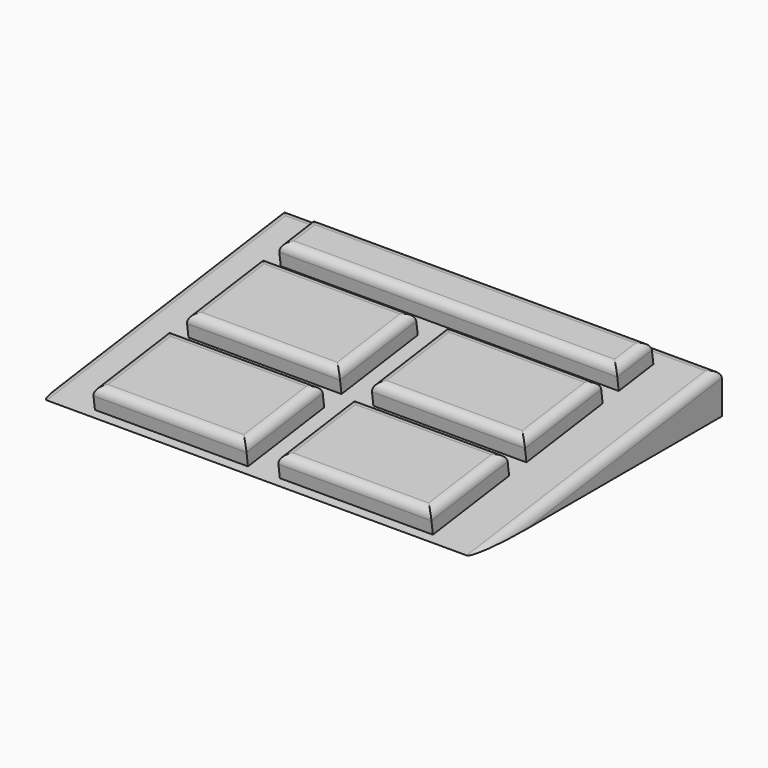
from build123d import *

# Parameters (mm, degrees)
F1_DEPTH  = 127
F2_R      = 5.08
F3_W      = 88.9
F3_H      = 55.88
F4_DEPTH  = 12.7
F5_R      = 5.08
F6_W      = 196.3208343999
F6_H      = 25.4
F7_DEPTH  = 12.7
F8_R      = 5.08
F9_R      = 8.0743885719
F10_DEPTH = 5.08


# Not quite as in the source:
# - a fillet or chamfer that OpenCascade refuses, or shapes differently, is made with other operations: its cross-section is extruded or revolved along the edge and cut away or added


with BuildPart() as f1:
    # F0 (on Right) → F1 (new body, symmetric)
    with BuildSketch(Plane.YZ):
        Polygon((102.2654771805, 0), (102.2654771805, 24.730855599), (-76.7904296517, 0), align=None)
    extrude(amount=F1_DEPTH, both=True)

    # F2
    f2_edges = [f1.edges().sort_by_distance(p)[0] for p in [
        (-127, 12.737524, 12.365428),
        (127, 12.737524, 12.365428),
        (0, 102.265477, 24.730856),
    ]]
    fillet(f2_edges, radius=F2_R)

    # F3 (on face) → F4 (join)
    with BuildSketch(Plane(origin=(0, -1.4374781315, 10.4076039488), x_dir=(1, 0, 0), z_dir=(0, -0.1368192087, 0.9905960348))):
        with Locations((-53.7104171999, 25.7286139321)):
            Rectangle(F3_W, F3_H)
        with Locations((53.7104171999, 25.7286139321)):
            Rectangle(F3_W, F3_H)
        with Locations((53.7104171999, -42.8513860679)):
            Rectangle(F3_W, F3_H)
        with Locations((-53.7104171999, -42.8513860679)):
            Rectangle(F3_W, F3_H)
    extrude(amount=F4_DEPTH)

    # F5
    f5_edges = [f1.edges().sort_by_distance(p)[0] for p in [
        (-98.160417, 22.311581, 26.508342),
        (-53.710417, -5.365672, 22.685613),
        (-98.160417, -45.623495, 17.125281),
        (-53.710417, -73.300748, 13.302552),
        (-53.710417, -17.946242, 20.94801),
        (-9.260417, -45.623495, 17.125281),
        (53.710417, -5.365672, 22.685613),
        (9.260417, 22.311581, 26.508342),
        (53.710417, 49.988834, 30.331071),
        (98.160417, 22.311581, 26.508342),
        (53.710417, -17.946242, 20.94801),
        (9.260417, -45.623495, 17.125281),
        (53.710417, -73.300748, 13.302552),
        (98.160417, -45.623495, 17.125281),
        (-9.260417, 22.311581, 26.508342),
        (-53.710417, 49.988834, 30.331071),
    ]]
    fillet(f5_edges, radius=F5_R)

    # F6 (on face) → F7 (join)
    with BuildSketch(Plane(origin=(0, -1.4374781315, 10.4076039488), x_dir=(1, 0, 0), z_dir=(0, -0.1368192087, 0.9905960348))):
        with Locations((0, 78.1313713312)):
            Rectangle(F6_W, F6_H)
    extrude(amount=F7_DEPTH)

    # F8
    f8_edges = [f1.edges().sort_by_distance(p)[0] for p in [
        (0, 61.640975, 31.940442),
        (0, 86.802114, 35.41565),
        (98.160417, 74.221545, 33.678046),
        (-98.160417, 74.221545, 33.678046),
    ]]
    fillet(f8_edges, radius=F8_R)

    # F9 (on face) → F10 (join)
    with BuildSketch(Plane(origin=(0, 0, 0), x_dir=(1, 0, 0), z_dir=(0, 0, -1))):
        with Locations((-114.6246567369, -91.883122921)):
            Circle(F9_R)
        with Locations((114.6246567369, -91.883122921)):
            Circle(F9_R)
    extrude(amount=F10_DEPTH)

    # F11: fillet of radius 7.62 on 2 edges, made by hand

    # F11_s1 → F11_t2 (revolve, cut)
    with BuildSketch(Plane.XZ.offset(-91.883122921)):
        with BuildLine():
            ThreePointArc((122.6990453088, 0), (119.9142494631, -3.6817039467), (115.5148404119, -5.08))
            Line((115.5148404119, -5.08), (122.6990453088, -5.08))
            Line((122.6990453088, -5.08), (122.6990453088, 0))
        make_face()
    revolve(axis=Axis((114.6246567369, 91.883122921, -5.08), (0, 0, -1)), mode=Mode.SUBTRACT)

    # F11_s3 → F11_t4 (revolve, cut)
    with BuildSketch(Plane.XZ.offset(-91.883122921)):
        with BuildLine():
            ThreePointArc((-106.5502681649, 0), (-109.3350640106, -3.6817039467), (-113.7344730618, -5.08))
            Line((-113.7344730618, -5.08), (-106.5502681649, -5.08))
            Line((-106.5502681649, -5.08), (-106.5502681649, 0))
        make_face()
    revolve(axis=Axis((-114.6246567369, 91.883122921, -5.08), (0, 0, -1)), mode=Mode.SUBTRACT)


solid = f1.part
